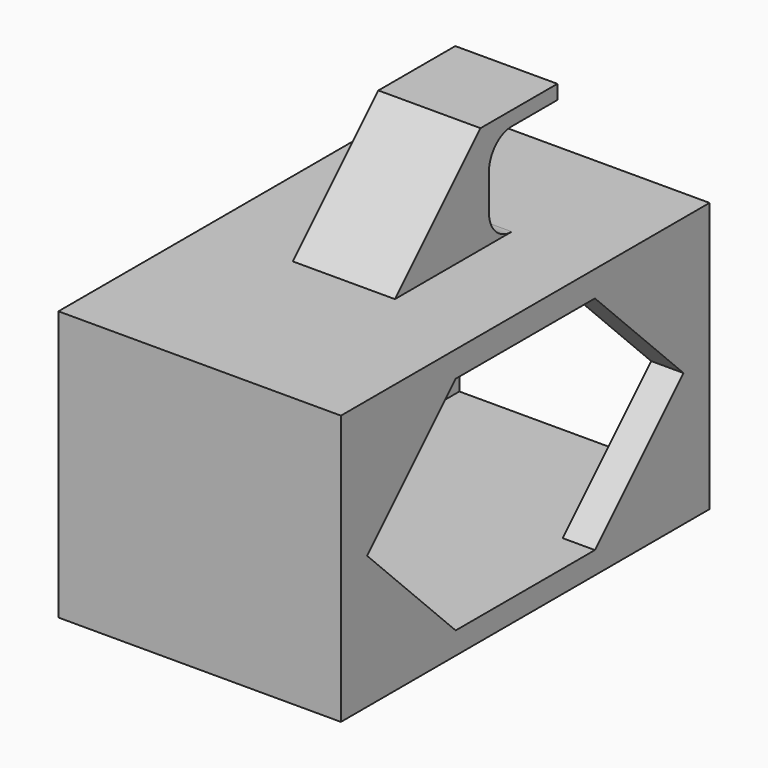
from build123d import *

# Parameters (mm, degrees)
F0_W          = 50.292
F0_H          = 82.042
F1_DEPTH      = 48.006
F2_W          = 39.4548750482
F2_H          = 39.4502789713
F3_DEPTH      = 101.6
F4_W          = 71.629058104
F4_H          = 39.4502789713
F5_DEPTH      = 101.6
F5_DEPTH_BACK = 25.4
F6_T1_DEPTH   = 5.7536101086
F6_T3_DEPTH   = 5.0835148431
F6_T8_DEPTH   = 58.0102084241
F6_T14_DEPTH  = 58.0102084241
F6_T20_DEPTH  = 58.0102084241
F6_T26_DEPTH  = 57.3401131586
F6_T32_DEPTH  = 57.3401131586
F6_T38_DEPTH  = 58.0102084241
F6_T44_DEPTH  = 57.3401131586
F6_T50_DEPTH  = 57.3401131586
F7_W          = 4.0118359902
F7_H          = 8.2200020552
F8_DEPTH      = 19.05
F9_DEPTH      = 12.7
F10_SIZE      = 19.04999
F11_DEPTH     = 5.08
F13_DEPTH     = 10.16
F14_W         = 18.1836719804
F14_H         = 16.51
F15_DEPTH     = 10.16
F16_R         = 5.08
F17_DEPTH     = 5.08
F18_W         = 38.7847797828
F18_H         = 3.7839086726
F19_DEPTH     = 40.64


# Not quite as in the source:
# - a fillet or chamfer that OpenCascade refuses, or shapes differently, is made with other operations: its cross-section is extruded or revolved along the edge and cut away or added
# - a fillet or chamfer is up to 0.001 mm smaller than in the source, because OpenCascade refuses the exact size


with BuildPart() as f1:
    # F0 (on Top) → F1 (new body)
    with BuildSketch(Plane.XY):
        with Locations((25.146, 41.021)):
            Rectangle(F0_W, F0_H)
    extrude(amount=F1_DEPTH)

    # F2 (on face) → F3 (cut)
    with BuildSketch(Plane.XZ):
        with Locations((24.8109523673, 23.683816893)):
            Rectangle(F2_W, F2_H)
    extrude(amount=-F3_DEPTH, mode=Mode.SUBTRACT)

    # F4 (on face) → F5 (cut, two sides)
    with BuildSketch(Plane.YZ.offset(5.0835148431)) as f5_sk:
        with Locations((41.033150861, 23.683816893)):
            Rectangle(F4_W, F4_H)
    extrude(amount=F5_DEPTH, mode=Mode.SUBTRACT)
    extrude(f5_sk.sketch, amount=-F5_DEPTH_BACK, mode=Mode.SUBTRACT)

    # F6: chamfer of 20.32 on 8 edges, made by hand

    # F6_s2 → F6_t1 (join)
    with BuildSketch(Plane.YZ.offset(44.5383898914)):
        Polygon((56.527679913, 3.9586774074), (76.847679913, 24.2786774074), (76.847679913, 3.9586774074), align=None)
        Polygon((25.538621809, 3.9586774074), (5.218621809, 24.2786774074), (5.218621809, 3.9586774074), align=None)
        Polygon((25.538621809, 43.4089563787), (5.218621809, 23.0889563787), (5.218621809, 43.4089563787), align=None)
        Polygon((56.527679913, 43.4089563787), (76.847679913, 23.0889563787), (76.847679913, 43.4089563787), align=None)
    extrude(amount=F6_T1_DEPTH)

    # F6_s4 → F6_t3 (join)
    with BuildSketch(Plane.YZ):
        Polygon((25.538621809, 43.4089563787), (5.218621809, 23.0889563787), (5.218621809, 43.4089563787), align=None)
        Polygon((25.538621809, 3.9586774074), (5.218621809, 24.2786774074), (5.218621809, 3.9586774074), align=None)
        Polygon((76.847679913, 23.0889563787), (56.527679913, 43.4089563787), (76.847679913, 43.4089563787), align=None)
        Polygon((56.527679913, 3.9586774074), (76.847679913, 24.2786774074), (76.847679913, 3.9586774074), align=None)
    extrude(amount=F6_T3_DEPTH)


with BuildPart() as f6_tool6:
    # F6_s7 → F6_t8 (new body)
    with BuildSketch(Plane.YZ.offset(-7.7182084241)):
        Polygon((56.527679913, 3.9586774074), (76.847679913, 24.2786774074), (76.847679913, 3.9586774074), align=None)
    extrude(amount=F6_T8_DEPTH)

    split(bisect_by=Plane.YZ, keep=Keep.TOP)

    split(bisect_by=Plane.YZ.offset(5.0835148431), keep=Keep.BOTTOM)


with BuildPart() as f1_1:
    add(f1.part)

    # F6_t5: union F6_tool6
    add(f6_tool6.part)


with BuildPart() as f6_tool12:
    # F6_s13 → F6_t14 (new body)
    with BuildSketch(Plane.YZ.offset(-7.7182084241)):
        Polygon((25.538621809, 3.9586774074), (5.218621809, 24.2786774074), (5.218621809, 3.9586774074), align=None)
    extrude(amount=F6_T14_DEPTH)

    split(bisect_by=Plane.YZ, keep=Keep.TOP)

    split(bisect_by=Plane.YZ.offset(5.0835148431), keep=Keep.BOTTOM)


with BuildPart() as f1_2:
    add(f1_1.part)

    # F6_t11: union F6_tool12
    add(f6_tool12.part)


with BuildPart() as f6_tool18:
    # F6_s19 → F6_t20 (new body)
    with BuildSketch(Plane.YZ.offset(50.292)):
        Polygon((25.538621809, 43.4089563787), (5.218621809, 23.0889563787), (5.218621809, 43.4089563787), align=None)
    extrude(amount=-F6_T20_DEPTH)

    split(bisect_by=Plane.YZ, keep=Keep.TOP)

    split(bisect_by=Plane.YZ.offset(5.0835148431), keep=Keep.BOTTOM)


with BuildPart() as f1_3:
    add(f1_2.part)

    # F6_t17: union F6_tool18
    add(f6_tool18.part)


with BuildPart() as f6_tool24:
    # F6_s25 → F6_t26 (new body)
    with BuildSketch(Plane.YZ.offset(57.3401131586)):
        Polygon((25.538621809, 43.4089563787), (5.218621809, 23.0889563787), (5.218621809, 43.4089563787), align=None)
    extrude(amount=-F6_T26_DEPTH)

    split(bisect_by=Plane.YZ.offset(50.292), keep=Keep.BOTTOM)

    split(bisect_by=Plane.YZ.offset(44.5383898914), keep=Keep.TOP)


with BuildPart() as f1_4:
    add(f1_3.part)

    # F6_t23: union F6_tool24
    add(f6_tool24.part)


with BuildPart() as f6_tool30:
    # F6_s31 → F6_t32 (new body)
    with BuildSketch(Plane.YZ):
        Polygon((25.538621809, 3.9586774074), (5.218621809, 24.2786774074), (5.218621809, 3.9586774074), align=None)
    extrude(amount=F6_T32_DEPTH)

    split(bisect_by=Plane.YZ.offset(50.292), keep=Keep.BOTTOM)

    split(bisect_by=Plane.YZ.offset(44.5383898914), keep=Keep.TOP)


with BuildPart() as f1_5:
    add(f1_4.part)

    # F6_t29: union F6_tool30
    add(f6_tool30.part)


with BuildPart() as f6_tool36:
    # F6_s37 → F6_t38 (new body)
    with BuildSketch(Plane.YZ.offset(50.292)):
        Polygon((56.527679913, 43.4089563787), (76.847679913, 23.0889563787), (76.847679913, 43.4089563787), align=None)
    extrude(amount=-F6_T38_DEPTH)

    split(bisect_by=Plane.YZ, keep=Keep.TOP)

    split(bisect_by=Plane.YZ.offset(5.0835148431), keep=Keep.BOTTOM)


with BuildPart() as f1_6:
    add(f1_5.part)

    # F6_t35: union F6_tool36
    add(f6_tool36.part)


with BuildPart() as f6_tool42:
    # F6_s43 → F6_t44 (new body)
    with BuildSketch(Plane.YZ.offset(57.3401131586)):
        Polygon((76.847679913, 23.0889563787), (56.527679913, 43.4089563787), (76.847679913, 43.4089563787), align=None)
    extrude(amount=-F6_T44_DEPTH)

    split(bisect_by=Plane.YZ.offset(50.292), keep=Keep.BOTTOM)

    split(bisect_by=Plane.YZ.offset(44.5383898914), keep=Keep.TOP)


with BuildPart() as f1_7:
    add(f1_6.part)

    # F6_t41: union F6_tool42
    add(f6_tool42.part)


with BuildPart() as f6_tool48:
    # F6_s49 → F6_t50 (new body)
    with BuildSketch(Plane.YZ):
        Polygon((56.527679913, 3.9586774074), (76.847679913, 24.2786774074), (76.847679913, 3.9586774074), align=None)
    extrude(amount=F6_T50_DEPTH)

    split(bisect_by=Plane.YZ.offset(50.292), keep=Keep.BOTTOM)

    split(bisect_by=Plane.YZ.offset(44.5383898914), keep=Keep.TOP)


with BuildPart() as f1_8:
    add(f1_7.part)

    # F6_t47: union F6_tool48
    add(f6_tool48.part)

    # F7 (on face) → F8 (join)
    with BuildSketch(Plane.XY.offset(48.006)):
        with Locations((27.1519179951, 36.1947827041)):
            Rectangle(F7_W, F7_H)
    extrude(amount=F8_DEPTH)

    # F9 (add): a face of the model
    f9_faces = [f1_8.faces().sort_by_distance(p)[0] for p in [
        (27.1519179951, 40.3047837317, 57.531),
    ]]
    extrude(f9_faces, amount=F9_DEPTH)

    # F10 (size 19.05 in the source; OpenCascade refuses exactly that, so slightly less here)
    f10_edges = [f1_8.edges().sort_by_distance(p)[0] for p in [
        (27.151918, 32.084782, 67.056),
    ]]
    chamfer(f10_edges, length=F10_SIZE)

    # F11 (add): a face of the model
    f11_faces = [f1_8.faces().sort_by_distance(p)[0] for p in [
        (29.1578359902, 45.9802990729, 54.8770427375),
    ]]
    extrude(f11_faces, amount=F11_DEPTH)

    # F12: F1 across face


with BuildPart() as f1_9:
    add(f1_8.part)
    add(f1_8.part.mirror(Plane(origin=(25.146, 45.9802990729, 54.8770427375), x_dir=(0, -1, 0), z_dir=(-1, 0, 0))))

    # F13 (add): a face of the model
    f13_faces = [f1_9.faces().sort_by_distance(p)[0] for p in [
        (25.146, 53.0047837317, 57.531),
    ]]
    extrude(f13_faces, amount=F13_DEPTH)

    # F14 (on face) → F15 (cut)
    with BuildSketch(Plane(origin=(0, 63.1647837317, 0), x_dir=(-1, 0, 0), z_dir=(0, 1, 0))):
        with Locations((-25.146, 56.261)):
            Rectangle(F14_W, F14_H)
    extrude(amount=-F15_DEPTH, mode=Mode.SUBTRACT)

    # F16
    f16_edges = [f1_9.edges().sort_by_distance(p)[0] for p in [
        (25.146, 53.004784, 64.516),
        (25.146, 53.004784, 48.006),
    ]]
    fillet(f16_edges, radius=F16_R)

    # F17 (add): a face of the model
    f17_faces = [f1_9.faces().sort_by_distance(p)[0] for p in [
        (25.146, 63.1647837317, 65.786),
    ]]
    extrude(f17_faces, amount=F17_DEPTH)

    # F18 (on face) → F19 (join)
    with BuildSketch(Plane.XY.offset(3.9586774074)):
        with Locations((25.146, 1.8919543363)):
            Rectangle(F18_W, F18_H)
    extrude(amount=F19_DEPTH)


solid = f1_9.part
